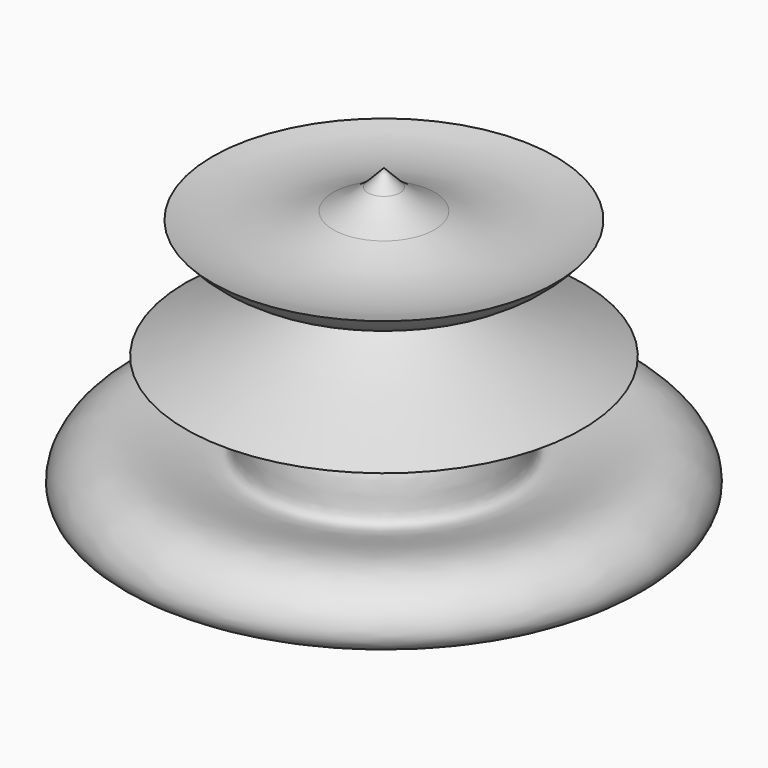
from build123d import *


with BuildPart() as f1:
    # F0 (on Front) → F1 (revolve)
    with BuildSketch(Plane.XZ):
        with BuildLine():
            add(Edge.make_bspline(
                [(0, 0), (-27.1051796503, -3.5443767226), (-67.4118240794, -8.7464089236), (-49.8728671609, 16.7989430499), (-22.8578637898, 0.9179825568), (-28.3916894921, 20.6344411436), (-11.2560722754, 23.9937113533), (-8.1846928224, 29.0724504739)],
                knots=[0, 0, 0, 0, 0.2368277581, 0.3510679428, 0.4979744028, 0.598423695, 0.738196034, 0.738196034, 0.738196034, 0.738196034], degree=3))
            Line((0, 0), (0, 62.0422624052))
            add(Edge.make_bspline(
                [(-8.1749800593, 48.3199730515), (-7.6130940571, 54.0499571493), (-3.5372618136, 58.377869456), (0, 62.0422624052)],
                knots=[0.8751966709, 0.8751966709, 0.8751966709, 0.8751966709, 1, 1, 1, 1], degree=3))
            add(Edge.make_bspline(
                [(-8.2085881563, 47.9179068994), (-8.1912557961, 48.0521851147), (-8.1800138349, 48.1862088062), (-8.1749800593, 48.3199730515)],
                knots=[0.5466905196, 0.5466905196, 0.5466905196, 0.5466905196, 0.5572633766, 0.5572633766, 0.5572633766, 0.5572633766], degree=3))
            add(Edge.make_bspline(
                [(-8.1846928224, 29.0724504739), (-5.2380080285, 33.9449983201), (-8.6414514377, 41.6931773133), (-8.2085881563, 47.9179068994)],
                knots=[0.738196034, 0.738196034, 0.738196034, 0.738196034, 0.8722937683, 0.8722937683, 0.8722937683, 0.8722937683], degree=3))
        make_face()
        with BuildLine():
            ThreePointArc((-43.4639267623, 25.7275477052), (-25.4443143414, 23.392125218), (-8.1846928224, 29.0724504739))
            add(Edge.make_bspline(
                [(-8.1846928224, 29.0724504739), (-5.2380080285, 33.9449983201), (-8.6414514377, 41.6931773133), (-8.2085881563, 47.9179068994)],
                knots=[0.738196034, 0.738196034, 0.738196034, 0.738196034, 0.8722937683, 0.8722937683, 0.8722937683, 0.8722937683], degree=3))
            add(Edge.make_bspline(
                [(-43.4639267623, 25.7275477052), (-26.2843594738, 33.3511667014), (-9.1047921853, 40.9747856976), (-8.2085881563, 47.9179068994)],
                knots=[0, 0, 0, 0, 0.5466905196, 0.5466905196, 0.5466905196, 0.5466905196], degree=3))
        make_face()
        with BuildLine():
            add(Edge.make_bspline(
                [(-8.1749800593, 48.3199730515), (-7.6130940571, 54.0499571493), (-3.5372618136, 58.377869456), (0, 62.0422624052)],
                knots=[0.8751966709, 0.8751966709, 0.8751966709, 0.8751966709, 1, 1, 1, 1], degree=3))
            Line((0, 62.0422624052), (-3.5372618136, 58.377869456))
            ThreePointArc((-3.5372618136, 58.377869456), (-7.1872518267, 55.8207072548), (-11.1179468634, 53.7204353325))
            add(Edge.make_bspline(
                [(-8.1749800593, 48.3199730515), (-8.1055853029, 50.1640237146), (-9.2160500863, 51.958766885), (-11.1179468634, 53.7204353325)],
                knots=[0.5572633766, 0.5572633766, 0.5572633766, 0.5572633766, 0.703018947, 0.703018947, 0.703018947, 0.703018947], degree=3))
        make_face()
        with BuildLine():
            ThreePointArc((-37.5822670758, 52.0133338869), (-23.6105035116, 44.3392771213), (-8.1749800593, 48.3199730515))
            add(Edge.make_bspline(
                [(-8.1749800593, 48.3199730515), (-8.1055853029, 50.1640237146), (-9.2160500863, 51.958766885), (-11.1179468634, 53.7204353325)],
                knots=[0.5572633766, 0.5572633766, 0.5572633766, 0.5572633766, 0.703018947, 0.703018947, 0.703018947, 0.703018947], degree=3))
            ThreePointArc((-11.1179468634, 53.7204353325), (-24.1920887828, 50.4172095152), (-37.5822670758, 52.0133338869))
        make_face()
    revolve(axis=Axis((0, 0, 31.0211312026), (0, 0, -1)))


solid = f1.part
